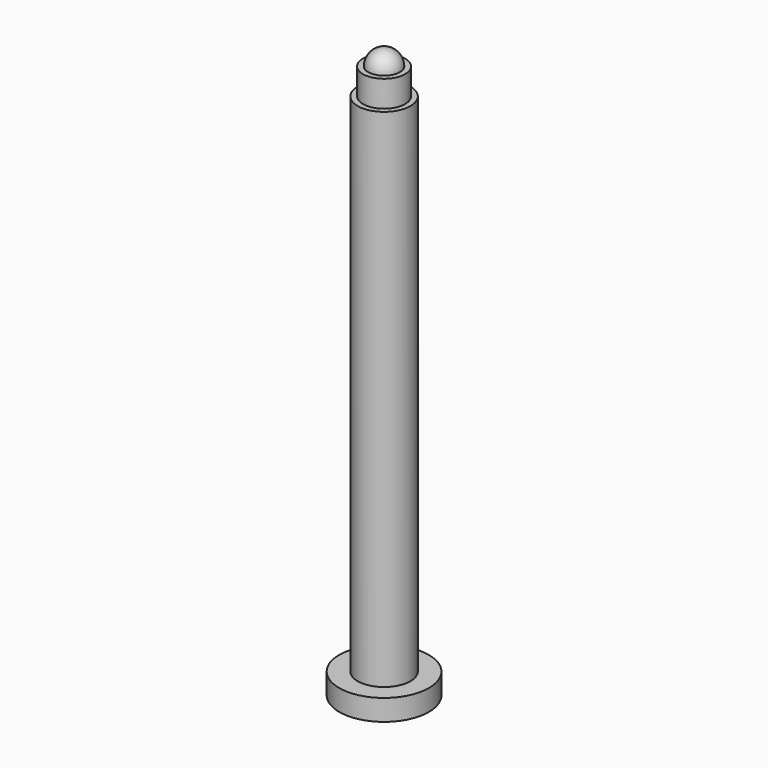
from build123d import *

# Parameters (mm, degrees)
F0_R         = 8.5
F1_DEPTH     = 4
F2_R         = 5
F3_DEPTH     = 100
F4_W         = 4
F4_H         = 5
F8_TEXT_SIZE = 9.9908055985
F9_DEPTH     = 0.1


# Not quite as in the source:
# - Text() gives the source's letters only with a copy of the font that has no kerning and outlines rounded to 1/6400 em; it was checked with that copy


with BuildPart() as f1:
    # F0 (on Top) → F1 (new body)
    with BuildSketch(Plane.XY):
        Circle(F0_R)
    extrude(amount=F1_DEPTH)

    # F2 (on Top) → F3 (join)
    with BuildSketch(Plane.XY):
        Circle(F2_R)
    extrude(amount=F3_DEPTH)

    # F4 (on Right) → F5 (revolve)
    with BuildSketch(Plane.YZ):
        with Locations((2, 102.5)):
            Rectangle(F4_W, F4_H)
    revolve(axis=Axis((0, 0, 102.5), (0, 0, -1)))

    # F6 (on Right) → F7 (revolve)
    with BuildSketch(Plane.YZ):
        with BuildLine():
            ThreePointArc((3, 105), (2.1213203436, 107.1213203436), (0, 108))
            Line((0, 108), (0, 105))
            Line((0, 105), (3, 105))
        make_face()
    revolve(axis=Axis((0, 0, 106.5), (0, 0, -1)))

    # F8 (on face) → F9 (cut)
    with BuildSketch(Plane(origin=(0, 0, 0), x_dir=(1, 0, 0), z_dir=(0, 0, -1))):
        with Locations((-7.712074625, -3.6193200177)):
            Text('E01', F8_TEXT_SIZE, font='Open Sans', text_align=(TextAlign.LEFT, TextAlign.BOTTOM))
    extrude(amount=-F9_DEPTH, mode=Mode.SUBTRACT)


solid = f1.part
